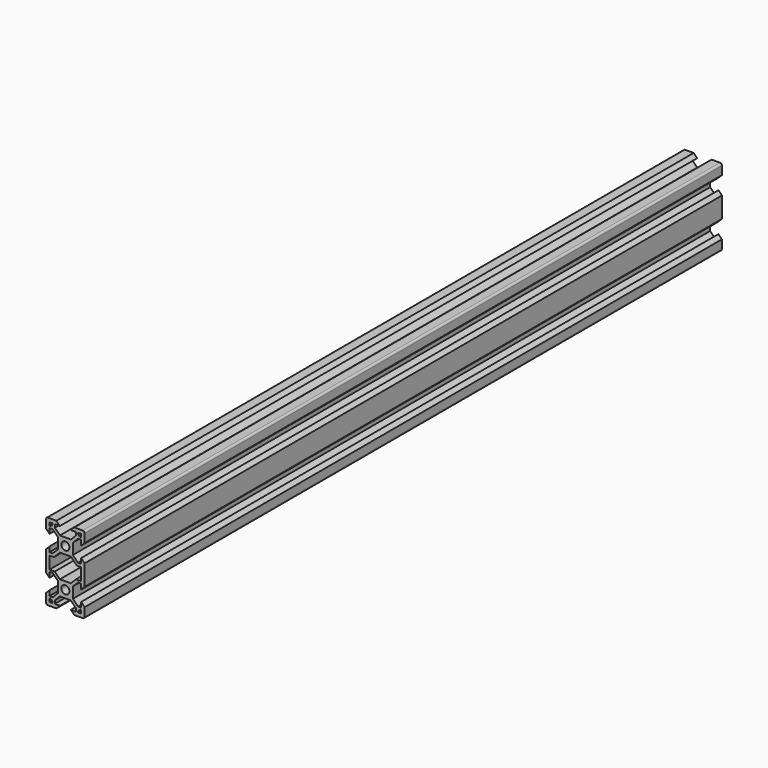
from build123d import *

# Parameters (mm, degrees)
F0_W             = 20
F0_H             = 20
F1_DEPTH         = 413
F2_R             = 2.1
F3_DEPTH         = 413.001
F4_R             = 1
F6_DEPTH         = 413.001
F6_COPIES3_COUNT = 2
F6_COPIES3_ANGLE = 90
F6_COPIES4_COUNT = 2
F6_COPIES4_ANGLE = 270
F6_COPIES6_COUNT = 2
F9_W             = 16.4
F9_H             = 6.8613203436
F10_DEPTH        = 413.001
F12_DEPTH        = 413


# Not quite as in the source:
# - a pattern or mirror of a feature is missing from the dataset's text; its kind, count and spacing are read off the source's solid


with BuildPart() as f1:
    # F0 (on Front) → F1 (new body)
    with BuildSketch(Plane.XZ):
        Rectangle(F0_W, F0_H)
    extrude(amount=F1_DEPTH)

    # F2 (on face) → F3 (cut, through all)
    with BuildSketch(Plane.XZ.offset(413)):
        Circle(F2_R)
    extrude(amount=-F3_DEPTH, mode=Mode.SUBTRACT)

    # F4
    f4_edges = [f1.edges().sort_by_distance(p)[0] for p in [
        (-10, -206.5, 10),
        (10, -206.5, 10),
    ]]
    fillet(f4_edges, radius=F4_R)

    # F5 (on face) → F6 (cut, through all)
    with BuildSketch(Plane.XZ.offset(413)):
        Polygon((0, 3.9006601718), (0, 10), (-2.84, 10), (-4.64, 10), (-2.84, 8.2), (-5.4993398282, 8.2), (-5.4993398282, 6.56), (-2.84, 3.9006601718), align=None)
        Polygon((-6.5693398282, 8.2), (-8.2, 8.2), (-7.0953059148, 7.0953059148), (-6.5693398282, 7.6212720014), align=None)
    f6 = extrude(amount=-F6_DEPTH, mode=Mode.SUBTRACT)

    # F6_copies: F6 across plane
    add(f6.mirror(Plane(origin=(0, 0, 0), x_dir=(-0.7071067812, 0, -0.7071067812), z_dir=(0.7071067812, 0, -0.7071067812))), mode=Mode.SUBTRACT)

    # F6_copies1: F6 across plane
    add(f6.mirror(Plane(origin=(0, 0, 0), x_dir=(0.7071067812, 0, -0.7071067812), z_dir=(-0.7071067812, 0, -0.7071067812))), mode=Mode.SUBTRACT)

    # F6_copies2: F6 across plane
    add(f6.mirror(Plane(origin=(0, 0, 0), x_dir=(0, 0, 1), z_dir=(1, 0, 0))), mode=Mode.SUBTRACT)

    # F6_copies3: F6 ×2 about axis
    f6_copies3_axis = Axis((0, 0, 0), (0, 1, 0))
    for i in range(1, F6_COPIES3_COUNT):
        add(f6.rotate(f6_copies3_axis, i * F6_COPIES3_ANGLE / (F6_COPIES3_COUNT - 1)), mode=Mode.SUBTRACT)

    # F6_copies4: F6 ×2 about axis
    f6_copies4_axis = Axis((0, 0, 0), (0, 1, 0))
    for i in range(1, F6_COPIES4_COUNT):
        add(f6.rotate(f6_copies4_axis, i * F6_COPIES4_ANGLE / (F6_COPIES4_COUNT - 1)), mode=Mode.SUBTRACT)

    # F6_copies5: F6 across plane
    add(f6.mirror(Plane(origin=(0, 0, 0), x_dir=(-1, 0, 0), z_dir=(0, 0, -1))), mode=Mode.SUBTRACT)

    # F6_copies6: F6 ×2 about axis
    f6_copies6_axis = Axis((0, 0, 0), (0, 1, 0))
    for i in range(1, F6_COPIES6_COUNT):
        add(f6.rotate(f6_copies6_axis, i * 360 / F6_COPIES6_COUNT), mode=Mode.SUBTRACT)

    # F8: F1 across face


with BuildPart() as f1_1:
    add(f1.part)
    add(f1.part.mirror(Plane(origin=(-7.32, -206.5, -10), x_dir=(1, 0, 0), z_dir=(0, 0, -1))))

    # F9 (on face) → F10 (cut, through all)
    with BuildSketch(Plane.XZ.offset(413)):
        with Locations((0, -10)):
            Rectangle(F9_W, F9_H)
    extrude(amount=-F10_DEPTH, mode=Mode.SUBTRACT)

    # F11 (on face) → F12 (join, through all)
    with BuildSketch(Plane.XZ.offset(413)):
        with BuildLine():
            ThreePointArc((-9, -10), (-9.7071067812, -9.7071067812), (-10, -9))
            Line((-10, -9), (-10, -11))
            ThreePointArc((-10, -11), (-9.7071067812, -10.2928932188), (-9, -10))
        make_face()
        with BuildLine():
            ThreePointArc((10, -9), (9.7071067812, -9.7071067812), (9, -10))
            ThreePointArc((9, -10), (9.7071067812, -10.2928932188), (10, -11))
            Line((10, -11), (10, -9))
        make_face()
        Polygon((5.9386796564, -6.9993398282), (8.2, -6.9993398282), (8.2, -6.5693398282), (5.5086796564, -6.5693398282), align=None)
        Polygon((-8.2, -6.5693398282), (-8.2, -6.9993398282), (-5.9386796564, -6.9993398282), (-5.5086796564, -6.5693398282), align=None)
    extrude(amount=-F12_DEPTH)


solid = f1_1.part
